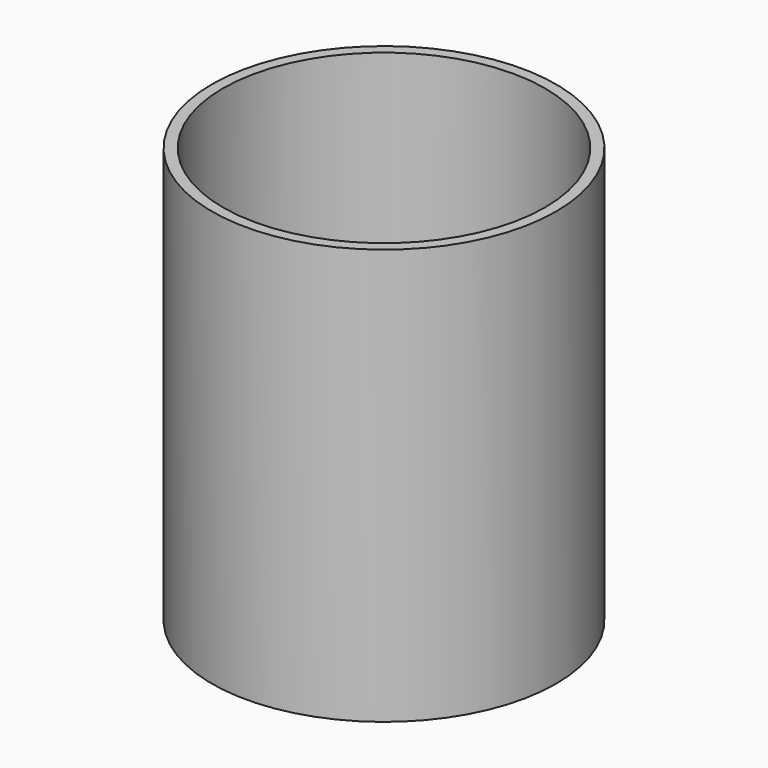
from build123d import *

# Parameters (mm, degrees)
F3_DEPTH = 25.4
F0_R     = 49.2232486947
F6_DEPTH = 25.4
F1_R     = 17.687795716
F0_R_2   = 52.5913484354
F7_DEPTH = 127
F9_DEPTH = 25


# Not quite as in the source:
# - a feature names something its author has since deleted; it is built from what else it names


with BuildPart() as f3:
    # F0 (on Top) → F3 (new body)
    with BuildSketch(Plane.XY):
        with BuildLine():
            ThreePointArc((-29.5833333333, -4.982608643), (-30, 0), (-29.5833333333, 4.982608643))
            ThreePointArc((-29.5833333333, 4.982608643), (-35, 0), (-29.5833333333, -4.982608643))
        make_face()
        with BuildLine():
            ThreePointArc((-25, 0), (-26.320099639, 3.3850160019), (-29.5833333333, 4.982608643))
            ThreePointArc((-29.5833333333, 4.982608643), (-30, 0), (-29.5833333333, -4.982608643))
            ThreePointArc((-29.5833333333, -4.982608643), (-26.320099639, -3.3850160019), (-25, 0))
        make_face()
    extrude(amount=F3_DEPTH)


with BuildPart() as f3b:
    # F0 (on Top) → F3, piece 2 (new body)
    with BuildSketch(Plane.XY):
        with BuildLine():
            ThreePointArc((-18.8360994911, -23.3495472325), (-15.8789717039, -25.4530598873), (-12.6894927419, -27.1841272428))
            ThreePointArc((-12.6894927419, -27.1841272428), (-15.3147928366, -24.5487142681), (-18.8360994911, -23.3495472325))
        make_face()
        with BuildLine():
            ThreePointArc((-11.4671403642, -31.4840823412), (-11.7786645812, -29.2489224373), (-12.6894927419, -27.1841272428))
            ThreePointArc((-12.6894927419, -27.1841272428), (-15.8789717039, -25.4530598873), (-18.8360994911, -23.3495472325))
            ThreePointArc((-18.8360994911, -23.3495472325), (-25.699594493, -36.9720742337), (-11.4671403642, -31.4840823412))
        make_face()
    extrude(amount=F3_DEPTH)


with BuildPart() as f3c:
    # F0 (on Top) → F3, piece 3 (new body)
    with BuildSketch(Plane.XY):
        with BuildLine():
            ThreePointArc((13.5205138222, -28.5316941921), (13.5108189409, -28.2447926413), (13.4817785281, -27.9592000205))
            ThreePointArc((13.4817785281, -27.9592000205), (12.6493579809, -29.63852128), (12.3268521898, -31.4848781997))
            ThreePointArc((12.3268521898, -31.4848781997), (13.2108144492, -30.1243432334), (13.5205138222, -28.5316941921))
        make_face()
        with BuildLine():
            ThreePointArc((25.4183405572, -31.6766425967), (20.8179668086, -25.4256248319), (13.4817785281, -27.9592000205))
            ThreePointArc((13.4817785281, -27.9592000205), (13.5108189409, -28.2447926413), (13.5205138222, -28.5316941921))
            ThreePointArc((13.5205138222, -28.5316941921), (13.2108144492, -30.1243432334), (12.3268521898, -31.4848781997))
            ThreePointArc((12.3268521898, -31.4848781997), (18.7752994046, -38.223088985), (25.4183405572, -31.6766425967))
        make_face()
    extrude(amount=F3_DEPTH)


with BuildPart() as f3d:
    # F0 (on Top) → F3, piece 4 (new body)
    with BuildSketch(Plane.XY):
        with BuildLine():
            ThreePointArc((30, 0), (29.9246449436, 2.125), (29.6989583333, 4.2393247003))
            ThreePointArc((29.6989583333, 4.2393247003), (25.75, 0), (29.6989583333, -4.2393247003))
            ThreePointArc((29.6989583333, -4.2393247003), (29.9246449436, -2.125), (30, 0))
        make_face()
        with BuildLine():
            ThreePointArc((29.6989583333, -4.2393247003), (32.8968148816, -3.1098172843), (34.25, 0))
            ThreePointArc((34.25, 0), (32.8968148816, 3.1098172843), (29.6989583333, 4.2393247003))
            ThreePointArc((29.6989583333, 4.2393247003), (29.9246449436, 2.125), (30, 0))
            ThreePointArc((30, 0), (29.9246449436, -2.125), (29.6989583333, -4.2393247003))
        make_face()
    extrude(amount=F3_DEPTH)


with BuildPart() as f6:
    # F0 (on Top) → F6 (new body)
    with BuildSketch(Plane.XY):
        Circle(F0_R)
        with BuildLine():
            ThreePointArc((29.6989583333, 4.2393247003), (32.8968148816, 3.1098172843), (34.25, 0))
            ThreePointArc((34.25, 0), (32.8968148816, -3.1098172843), (29.6989583333, -4.2393247003))
            ThreePointArc((29.6989583333, -4.2393247003), (24.2705110645, -17.6335558713), (13.2093239888, -26.9353626253))
            ThreePointArc((13.2093239888, -26.9353626253), (13.3775797895, -27.4387581739), (13.4817785281, -27.9592000205))
            ThreePointArc((13.4817785281, -27.9592000205), (20.8179668086, -25.4256248319), (25.4183405572, -31.6766425967))
            ThreePointArc((25.4183405572, -31.6766425967), (18.7752994046, -38.223088985), (12.3268521898, -31.4848781997))
            ThreePointArc((12.3268521898, -31.4848781997), (8.1677226938, -32.6361249355), (5.1456495934, -29.5554105074))
            ThreePointArc((5.1456495934, -29.5554105074), (-3.9538763818, -29.7383062994), (-12.6894927419, -27.1841272428))
            ThreePointArc((-12.6894927419, -27.1841272428), (-11.7786645812, -29.2489224373), (-11.4671403642, -31.4840823412))
            ThreePointArc((-11.4671403642, -31.4840823412), (-25.699594493, -36.9720742337), (-18.8360994911, -23.3495472325))
            ThreePointArc((-18.8360994911, -23.3495472325), (-20.2231622396, -22.1590547865), (-21.5351472772, -20.8862977032))
            ThreePointArc((-21.5351472772, -20.8862977032), (-27.7088299454, -20.1316477979), (-26.5187730739, -14.0269267715))
            ThreePointArc((-26.5187730739, -14.0269267715), (-28.4132277018, -9.6274862537), (-29.5833333333, -4.982608643))
            ThreePointArc((-29.5833333333, -4.982608643), (-35, 0), (-29.5833333333, 4.982608643))
            ThreePointArc((-29.5833333333, 4.982608643), (-28.4132285435, 9.6274837697), (-26.5187755265, 14.0269221349))
            ThreePointArc((-26.5187755265, 14.0269221349), (-27.7088334653, 20.1316429531), (-21.5351509291, 20.8862939379))
            ThreePointArc((-21.5351509291, 20.8862939379), (-9.2705113278, 28.5316950026), (5.1456444258, 29.5554114071))
            ThreePointArc((5.1456444258, 29.5554114071), (9.7861764915, 32.7502959205), (13.5205088335, 28.531695813))
            ThreePointArc((13.5205088335, 28.531695813), (13.4419860536, 27.7185059196), (13.2093192793, 26.9353649349))
            ThreePointArc((13.2093192793, 26.9353649349), (24.2705095229, 17.6335579931), (29.6989583333, 4.2393247003))
        make_face(mode=Mode.SUBTRACT)
    extrude(amount=F6_DEPTH)

    # F0 (on Top) → F7 (join)
    with BuildSketch(Plane.XY):
        Circle(F0_R_2)
        Circle(F0_R, mode=Mode.SUBTRACT)
    extrude(amount=F7_DEPTH)


with BuildPart() as f6b:
    # F1 (on Top) → F6, piece 2 (new body)
    with BuildSketch(Plane.XY):
        Circle(F1_R)
    extrude(amount=F6_DEPTH)

    # F0 (on Top) → F9 (join)
    with BuildSketch(Plane.XY):
        Circle(F0_R)
        with BuildLine():
            ThreePointArc((29.6989583333, 4.2393247003), (32.8968148816, 3.1098172843), (34.25, 0))
            ThreePointArc((34.25, 0), (32.8968148816, -3.1098172843), (29.6989583333, -4.2393247003))
            ThreePointArc((29.6989583333, -4.2393247003), (24.2705110645, -17.6335558713), (13.2093239888, -26.9353626253))
            ThreePointArc((13.2093239888, -26.9353626253), (13.3775797895, -27.4387581739), (13.4817785281, -27.9592000205))
            ThreePointArc((13.4817785281, -27.9592000205), (20.8179668086, -25.4256248319), (25.4183405572, -31.6766425967))
            ThreePointArc((25.4183405572, -31.6766425967), (18.7752994046, -38.223088985), (12.3268521898, -31.4848781997))
            ThreePointArc((12.3268521898, -31.4848781997), (8.1677226938, -32.6361249355), (5.1456495934, -29.5554105074))
            ThreePointArc((5.1456495934, -29.5554105074), (-3.9538763818, -29.7383062994), (-12.6894927419, -27.1841272428))
            ThreePointArc((-12.6894927419, -27.1841272428), (-11.7786645812, -29.2489224373), (-11.4671403642, -31.4840823412))
            ThreePointArc((-11.4671403642, -31.4840823412), (-25.699594493, -36.9720742337), (-18.8360994911, -23.3495472325))
            ThreePointArc((-18.8360994911, -23.3495472325), (-20.2231622396, -22.1590547865), (-21.5351472772, -20.8862977032))
            ThreePointArc((-21.5351472772, -20.8862977032), (-27.7088299454, -20.1316477979), (-26.5187730739, -14.0269267715))
            ThreePointArc((-26.5187730739, -14.0269267715), (-28.4132277018, -9.6274862537), (-29.5833333333, -4.982608643))
            ThreePointArc((-29.5833333333, -4.982608643), (-35, 0), (-29.5833333333, 4.982608643))
            ThreePointArc((-29.5833333333, 4.982608643), (-28.4132285435, 9.6274837697), (-26.5187755265, 14.0269221349))
            ThreePointArc((-26.5187755265, 14.0269221349), (-27.7088334653, 20.1316429531), (-21.5351509291, 20.8862939379))
            ThreePointArc((-21.5351509291, 20.8862939379), (-9.2705113278, 28.5316950026), (5.1456444258, 29.5554114071))
            ThreePointArc((5.1456444258, 29.5554114071), (9.7861764915, 32.7502959205), (13.5205088335, 28.531695813))
            ThreePointArc((13.5205088335, 28.531695813), (13.4419860536, 27.7185059196), (13.2093192793, 26.9353649349))
            ThreePointArc((13.2093192793, 26.9353649349), (24.2705095229, 17.6335579931), (29.6989583333, 4.2393247003))
        make_face(mode=Mode.SUBTRACT)
        with BuildLine():
            ThreePointArc((29.6989583333, -4.2393247003), (25.75, 0), (29.6989583333, 4.2393247003))
            ThreePointArc((29.6989583333, 4.2393247003), (24.2705095229, 17.6335579931), (13.2093192793, 26.9353649349))
            ThreePointArc((13.2093192793, 26.9353649349), (7.9571867488, 24.4897055729), (5.1456444258, 29.5554114071))
            ThreePointArc((5.1456444258, 29.5554114071), (-9.2705113278, 28.5316950026), (-21.5351509291, 20.8862939379))
            ThreePointArc((-21.5351509291, 20.8862939379), (-20.4177341066, 19.4276042855), (-20.0205110645, 17.6335558713))
            ThreePointArc((-20.0205110645, 17.6335558713), (-22.2080639698, 13.9175348836), (-26.5187755265, 14.0269221349))
            ThreePointArc((-26.5187755265, 14.0269221349), (-28.4132285435, 9.6274837697), (-29.5833333333, 4.982608643))
            ThreePointArc((-29.5833333333, 4.982608643), (-26.320099639, 3.3850160019), (-25, 0))
            ThreePointArc((-25, 0), (-26.320099639, -3.3850160019), (-29.5833333333, -4.982608643))
            ThreePointArc((-29.5833333333, -4.982608643), (-28.4132277018, -9.6274862537), (-26.5187730739, -14.0269267715))
            ThreePointArc((-26.5187730739, -14.0269267715), (-22.2080612115, -13.9175389468), (-20.0205079814, -17.6335601149))
            ThreePointArc((-20.0205079814, -17.6335601149), (-20.4177308666, -19.4276081922), (-21.5351472772, -20.8862977032))
            ThreePointArc((-21.5351472772, -20.8862977032), (-20.2231622396, -22.1590547865), (-18.8360994911, -23.3495472325))
            ThreePointArc((-18.8360994911, -23.3495472325), (-15.3147928366, -24.5487142681), (-12.6894927419, -27.1841272428))
            ThreePointArc((-12.6894927419, -27.1841272428), (-3.9538763818, -29.7383062994), (5.1456495934, -29.5554105074))
            ThreePointArc((5.1456495934, -29.5554105074), (7.9571910307, -24.4897041816), (13.2093239888, -26.9353626253))
            ThreePointArc((13.2093239888, -26.9353626253), (24.2705110645, -17.6335558713), (29.6989583333, -4.2393247003))
        make_face()
    extrude(amount=F9_DEPTH)


solid = Compound([f3.part, f3b.part, f3c.part, f3d.part, f6.part, f6b.part])
